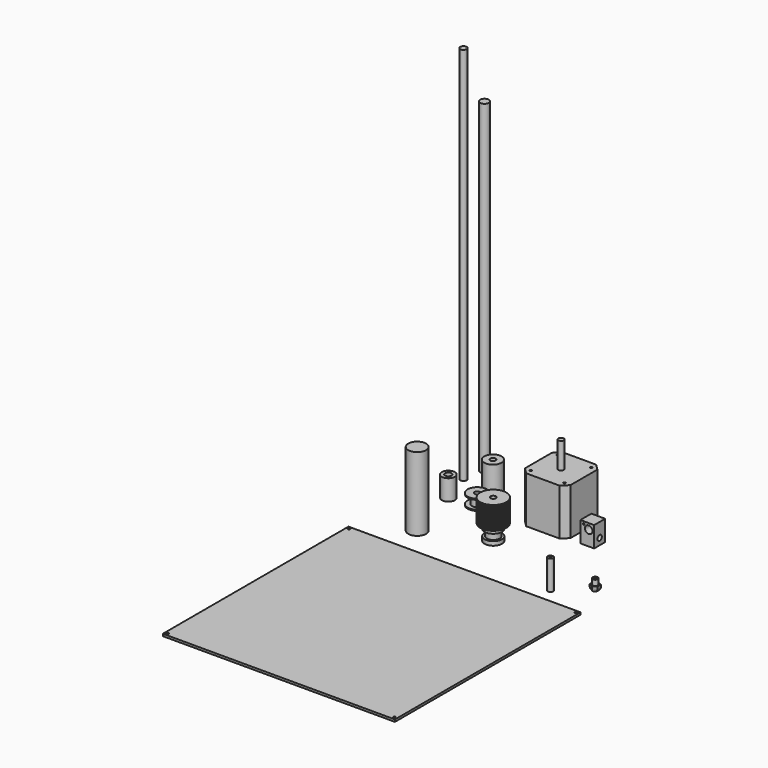
from build123d import *

# Parameters (mm, degrees)
F0_R         = 3
F1_DEPTH     = 350
F2_R         = 8
F2_R_2       = 4
F3_DEPTH     = 25
F4_R         = 6
F4_R_2       = 3
F5_DEPTH     = 19
F6_R         = 5
F7_DEPTH     = 10
F8_R         = 9
F8_R_2       = 5
F9_DEPTH     = 1
F10_R        = 9
F11_DEPTH    = 1
F12_R        = 1
F12_R_2      = 2.5
F13_DEPTH    = 43
F14_DEPTH    = 67
F15_R        = 4
F15_R_2      = 2.5
F16_DEPTH    = 12
F17_R        = 4
F18_DEPTH    = 300
F19_W        = 214
F19_H        = 214
F19_R        = 1
F20_DEPTH    = 2
F21_R        = 8.25
F22_DEPTH    = 68
F23_R        = 2
F24_DEPTH    = 1.7
F25_R        = 8
F25_R_2      = 2
F26_DEPTH    = 3.7
F27_R        = 6
F28_DEPTH    = 6
F29_R        = 8
F29_R_2      = 6
F30_DEPTH    = 3
F31_R        = 4
F32_DEPTH    = 6
F33_R        = 5
F34_DEPTH    = 1.5
F35_R        = 12
F36_DEPTH    = 1
F37_R        = 5
F38_DEPTH    = 1.5
F39_R        = 12
F40_DEPTH    = 1
F41_R        = 5
F42_DEPTH    = 1.5
F43_R        = 12
F44_DEPTH    = 1
F45_R        = 5.5
F46_DEPTH    = 1.5
F47_R        = 12
F48_DEPTH    = 1
F49_R        = 5.5
F50_DEPTH    = 1.5
F51_R        = 12
F52_DEPTH    = 1
F53_R        = 5.5
F54_DEPTH    = 1.5
F55_R        = 12
F56_DEPTH    = 1
F57_R        = 5.5
F58_DEPTH    = 1.5
F59_R        = 12
F60_DEPTH    = 1
F61_R        = 5.5
F62_DEPTH    = 1.5
F63_R        = 12
F64_DEPTH    = 1
F65_R        = 5.5
F66_DEPTH    = 1.5
F67_R        = 12
F67_R_2      = 5.5
F68_DEPTH    = 1
F69_R        = 0.875
F70_DEPTH    = 63
F71_R        = 2.5
F71_R_2      = 0.875
F72_DEPTH    = 15
F73_W        = 12.7
F73_H        = 19
F73_R        = 0.75
F73_R_2      = 3.5
F74_DEPTH    = 12.7
F75_R        = 2.5
F76_DEPTH    = 25
F77_R        = 0.1
F78_DEPTH    = 5
F79_T1_DEPTH = 19.975261396
F79_T3_DEPTH = 19.975261396
F79_T5_DEPTH = 19.975261396
F79_T7_DEPTH = 19.975261396
F79_T9_DEPTH = 19.975261396
F80_R        = 0.875
F81_DEPTH    = 3.04
F82_R        = 2.5
F82_R_2      = 0.875
F83_DEPTH    = 5
F84_R        = 2.5
F84_R_2      = 0.875
F85_DEPTH    = 27
F86_R        = 2.5
F87_DEPTH    = 25


# Not quite as in the source:
# - a fillet or chamfer that OpenCascade refuses, or shapes differently, is made with other operations: its cross-section is extruded or revolved along the edge and cut away or added


with BuildPart() as f1:
    # F0 (on Top) → F1 (new body)
    with BuildSketch(Plane.XY):
        with Locations((-57.2636425495, 36.8765890598)):
            Circle(F0_R)
    extrude(amount=F1_DEPTH)


with BuildPart() as f3:
    # F2 (on Top) → F3 (new body)
    with BuildSketch(Plane.XY):
        with Locations((-29.7810900956, 36.4768393338)):
            Circle(F2_R)
        with Locations((-29.7810900956, 36.4768393338)):
            Circle(F2_R_2, mode=Mode.SUBTRACT)
    extrude(amount=F3_DEPTH)

    # F15 (on face) → F16 (join)
    with BuildSketch(Plane.XY.offset(25)):
        with Locations((-29.7810900956, 36.4768393338)):
            Circle(F15_R)
        with Locations((-29.7810900956, 36.4768393338)):
            Circle(F15_R_2, mode=Mode.SUBTRACT)
    extrude(amount=-F16_DEPTH)


with BuildPart() as f5:
    # F4 (on Top) → F5 (new body)
    with BuildSketch(Plane.XY):
        with Locations((-47.5174151361, 7.268529851)):
            Circle(F4_R)
        with Locations((-47.5174151361, 7.268529851)):
            Circle(F4_R_2, mode=Mode.SUBTRACT)
    extrude(amount=F5_DEPTH)


with BuildPart() as f7:
    # F6 (on Top) → F7 (new body)
    with BuildSketch(Plane.XY):
        with Locations((-24.0222588181, 11.2928301096)):
            Circle(F6_R)
    extrude(amount=F7_DEPTH)

    # F8 (on face) → F9 (join)
    with BuildSketch(Plane.XY.offset(10)):
        with Locations((-24.0222588181, 11.2928301096)):
            Circle(F8_R)
        with Locations((-24.0222588181, 11.2928301096)):
            Circle(F8_R_2, mode=Mode.SUBTRACT)
    extrude(amount=-F9_DEPTH)

    # F10 (on face) → F11 (join)
    with BuildSketch(Plane(origin=(0, 0, 0), x_dir=(1, 0, 0), z_dir=(0, 0, -1))):
        with Locations((-24.0552949804, -11.3842185209)):
            Circle(F10_R)
    extrude(amount=-F11_DEPTH)

    # F86 (on face) → F87 (cut)
    with BuildSketch(Plane.XY.offset(10)):
        with Locations((-24.0222588181, 11.2928301096)):
            Circle(F86_R)
    extrude(amount=-F87_DEPTH, mode=Mode.SUBTRACT)


with BuildPart() as f13:
    # F12 (on Top) → F13 (new body)
    with BuildSketch(Plane.XY):
        Polygon((54.8616796434, 49.6951151714), (23.8616796434, 49.6951151714), (18.3616796434, 44.1951151714), (18.3616796434, 13.1951151714), (23.8616796434, 7.6951151714), (54.8616796434, 7.6951151714), (60.3616796434, 13.1951151714), (60.3616796434, 44.1951151714), align=None)
        with Locations((23.8616796434, 13.1951151714)):
            Circle(F12_R, mode=Mode.SUBTRACT)
        with Locations((54.8616796434, 13.1951151714)):
            Circle(F12_R, mode=Mode.SUBTRACT)
        with Locations((23.8616796434, 44.1951151714)):
            Circle(F12_R, mode=Mode.SUBTRACT)
        with Locations((39.3616796434, 28.6951151714)):
            Circle(F12_R_2, mode=Mode.SUBTRACT)
        with Locations((54.8616796434, 44.1951151714)):
            Circle(F12_R, mode=Mode.SUBTRACT)
    extrude(amount=F13_DEPTH)

    # F12 (on Top) → F14 (join)
    with BuildSketch(Plane.XY):
        with Locations((39.3616796434, 28.6951151714)):
            Circle(F12_R_2)
    extrude(amount=F14_DEPTH)


with BuildPart() as f18:
    # F17 (on Top) → F18 (new body)
    with BuildSketch(Plane.XY):
        with Locations((-53.5317584872, 56.4855635166)):
            Circle(F17_R)
    extrude(amount=F18_DEPTH)


with BuildPart() as f20:
    # F19 (on Top) → F20 (new body)
    with BuildSketch(Plane.XY):
        with Locations((33.727236867, -182.6495461464)):
            Rectangle(F19_W, F19_H)
        with Locations((-70.772763133, -287.1495461464)):
            Circle(F19_R, mode=Mode.SUBTRACT)
        with Locations((138.227236867, -287.1495461464)):
            Circle(F19_R, mode=Mode.SUBTRACT)
        with Locations((-70.772763133, -78.1495461464)):
            Circle(F19_R, mode=Mode.SUBTRACT)
        with Locations((138.227236867, -78.1495461464)):
            Circle(F19_R, mode=Mode.SUBTRACT)
    extrude(amount=F20_DEPTH)


with BuildPart() as f22:
    # F21 (on Top) → F22 (new body)
    with BuildSketch(Plane.XY):
        with Locations((-33.137626946, -46.6584786773)):
            Circle(F21_R)
    extrude(amount=F22_DEPTH)


with BuildPart() as f24:
    # F23 (on Top) → F24 (new body)
    with BuildSketch(Plane.XY):
        with Locations((21.4881356806, -27.2024124861)):
            Circle(F23_R)
    extrude(amount=F24_DEPTH)

    # F25 (on face) → F26 (join)
    with BuildSketch(Plane.XY.offset(1.7)):
        with Locations((21.4881356806, -27.2024124861)):
            Circle(F25_R)
        with Locations((21.4881356806, -27.2024124861)):
            Circle(F25_R_2, mode=Mode.SUBTRACT)
        with Locations((21.4881356806, -27.2024124861)):
            Circle(F25_R_2)
    extrude(amount=F26_DEPTH)

    # F27 (on face) → F28 (join)
    with BuildSketch(Plane.XY.offset(5.4)):
        with Locations((21.4881356806, -27.2024124861)):
            Circle(F27_R)
    extrude(amount=F28_DEPTH)

    # F29 (on face) → F30 (join)
    with BuildSketch(Plane.XY.offset(11.4)):
        with Locations((21.4881356806, -27.2024124861)):
            Circle(F29_R)
        with Locations((21.4881356806, -27.2024124861)):
            Circle(F29_R_2, mode=Mode.SUBTRACT)
        with Locations((21.4881356806, -27.2024124861)):
            Circle(F29_R_2)
    extrude(amount=F30_DEPTH)

    # F31 (on face) → F32 (cut)
    with BuildSketch(Plane(origin=(0, 0, 0), x_dir=(1, 0, 0), z_dir=(0, 0, -1))):
        with Locations((21.4881356806, 27.2024124861)):
            Circle(F31_R)
    extrude(amount=-F32_DEPTH, mode=Mode.SUBTRACT)

    # F33 (on face) → F34 (join)
    with BuildSketch(Plane.XY.offset(14.4)):
        with Locations((21.4881356806, -27.2024124861)):
            Circle(F33_R)
    extrude(amount=F34_DEPTH)

    # F35 (on face) → F36 (join)
    with BuildSketch(Plane.XY.offset(15.9)):
        with Locations((21.4881356806, -27.2024124861)):
            Circle(F35_R)
    extrude(amount=F36_DEPTH)

    # F37 (on face) → F38 (join)
    with BuildSketch(Plane.XY.offset(16.9)):
        with Locations((21.4881356806, -27.2024124861)):
            Circle(F37_R)
    extrude(amount=F38_DEPTH)

    # F39 (on face) → F40 (join)
    with BuildSketch(Plane.XY.offset(18.4)):
        with Locations((21.4881356806, -27.2024124861)):
            Circle(F39_R)
    extrude(amount=F40_DEPTH)

    # F41 (on face) → F42 (join)
    with BuildSketch(Plane.XY.offset(19.4)):
        with Locations((21.4881356806, -27.2024124861)):
            Circle(F41_R)
    extrude(amount=F42_DEPTH)

    # F43 (on face) → F44 (join)
    with BuildSketch(Plane.XY.offset(20.9)):
        with Locations((21.4881356806, -27.2024124861)):
            Circle(F43_R)
    extrude(amount=F44_DEPTH)

    # F45 (on face) → F46 (join)
    with BuildSketch(Plane.XY.offset(21.9)):
        with Locations((21.4881356806, -27.2024124861)):
            Circle(F45_R)
    extrude(amount=F46_DEPTH)

    # F47 (on face) → F48 (join)
    with BuildSketch(Plane.XY.offset(23.4)):
        with Locations((21.4881356806, -27.2024124861)):
            Circle(F47_R)
    extrude(amount=F48_DEPTH)

    # F49 (on face) → F50 (join)
    with BuildSketch(Plane.XY.offset(24.4)):
        with Locations((21.4881356806, -27.2024124861)):
            Circle(F49_R)
    extrude(amount=F50_DEPTH)

    # F51 (on face) → F52 (join)
    with BuildSketch(Plane.XY.offset(25.9)):
        with Locations((21.4881356806, -27.2024124861)):
            Circle(F51_R)
    extrude(amount=F52_DEPTH)

    # F53 (on face) → F54 (join)
    with BuildSketch(Plane.XY.offset(26.9)):
        with Locations((21.4881356806, -27.2024124861)):
            Circle(F53_R)
    extrude(amount=F54_DEPTH)

    # F55 (on face) → F56 (join)
    with BuildSketch(Plane.XY.offset(28.4)):
        with Locations((21.4881356806, -27.2024124861)):
            Circle(F55_R)
    extrude(amount=F56_DEPTH)

    # F57 (on face) → F58 (join)
    with BuildSketch(Plane.XY.offset(29.4)):
        with Locations((21.4881356806, -27.2024124861)):
            Circle(F57_R)
    extrude(amount=F58_DEPTH)

    # F59 (on face) → F60 (join)
    with BuildSketch(Plane.XY.offset(30.9)):
        with Locations((21.4881356806, -27.2024124861)):
            Circle(F59_R)
    extrude(amount=F60_DEPTH)

    # F61 (on face) → F62 (join)
    with BuildSketch(Plane.XY.offset(31.9)):
        with Locations((21.4881356806, -27.2024124861)):
            Circle(F61_R)
    extrude(amount=F62_DEPTH)

    # F63 (on face) → F64 (join)
    with BuildSketch(Plane.XY.offset(33.4)):
        with Locations((21.4881356806, -27.2024124861)):
            Circle(F63_R)
    extrude(amount=F64_DEPTH)

    # F65 (on face) → F66 (join)
    with BuildSketch(Plane.XY.offset(34.4)):
        with Locations((21.4881356806, -27.2024124861)):
            Circle(F65_R)
    extrude(amount=F66_DEPTH)

    # F67 (on face) → F68 (join)
    with BuildSketch(Plane.XY.offset(35.9)):
        with Locations((21.4881356806, -27.2024124861)):
            Circle(F67_R)
        with Locations((21.4881356806, -27.2024124861)):
            Circle(F67_R_2, mode=Mode.SUBTRACT)
        with Locations((21.4881356806, -27.2024124861)):
            Circle(F67_R_2)
    extrude(amount=F68_DEPTH)

    # F69 (on face) → F70 (cut)
    with BuildSketch(Plane(origin=(0, 0, 6), x_dir=(1, 0, 0), z_dir=(0, 0, -1))):
        with Locations((21.4881356806, 27.2024124861)):
            Circle(F69_R)
    extrude(amount=-F70_DEPTH, mode=Mode.SUBTRACT)

    # F71 (on face) → F72 (cut)
    with BuildSketch(Plane.XY.offset(36.9)):
        with Locations((21.4881356806, -27.2024124861)):
            Circle(F71_R)
        with Locations((21.4881356806, -27.2024124861)):
            Circle(F71_R_2, mode=Mode.SUBTRACT)
    extrude(amount=-F72_DEPTH, mode=Mode.SUBTRACT)


with BuildPart() as f74:
    # F73 (on Front) → F74 (new body)
    with BuildSketch(Plane.XZ):
        with Locations((96.546877718, 25.4235037863)):
            Rectangle(F73_W, F73_H)
        with Locations((93.1878611445, 32.6125212014)):
            Circle(F73_R, mode=Mode.SUBTRACT)
        with Locations((97.896877718, 29.5235037863)):
            Circle(F73_R_2, mode=Mode.SUBTRACT)
    extrude(amount=F74_DEPTH)

    # F75 (on face) → F76 (cut)
    with BuildSketch(Plane(origin=(90.196877718, 0, 0), x_dir=(0, -1, 0), z_dir=(-1, 0, 0))):
        with Locations((6.35, 21.9235037863)):
            Circle(F75_R)
    extrude(amount=-F76_DEPTH, mode=Mode.SUBTRACT)


with BuildPart() as f78:
    # F77 (on Top) → F78 (new body)
    with BuildSketch(Plane.XY):
        Polygon((121.874764204, -37.4743435914), (121.874764204, -41.5157954758), (125.374764204, -43.5365214179), (128.874764204, -41.5157954758), (128.874764204, -37.4743435914), (125.374764204, -35.4536176493), align=None)
        with Locations((125.374764204, -39.4950695336)):
            Circle(F77_R, mode=Mode.SUBTRACT)
    extrude(amount=F78_DEPTH)

    # F79: fillet of radius 3.1867619023 on 6 edges, made by hand

    # F79_s2 → F79_t1 (cut)
    with BuildSketch(Plane(origin=(85.5787482909, 49.4089133627, 0), x_dir=(0, 0, 1), z_dir=(-0.8660254038, -0.5, 0))):
        with BuildLine():
            add(Edge.make_bspline(
                [(3.1867619023, -93.3911156423), (0, -93.3911156423), (0, -96.5778775447)],
                knots=[0, 0, 0, 1, 1, 1], degree=2, weights=[1, 1, 1]))
            Line((0, -96.5778775447), (0, -93.3911156423))
            Line((0, -93.3911156423), (3.1867619023, -93.3911156423))
        make_face()
    extrude(amount=F79_T1_DEPTH, mode=Mode.SUBTRACT)

    # F79_s4 → F79_t3 (cut)
    with BuildSketch(Plane.XZ.offset(29.5074388356)):
        with BuildLine():
            add(Edge.make_bspline(
                [(121.874764204, 3.1867619023), (121.874764204, 0), (125.0615261064, 0)],
                knots=[0, 0, 0, 1, 1, 1], degree=2, weights=[1, 1, 1]))
            Line((125.0615261064, 0), (121.874764204, 0))
            Line((121.874764204, 0), (121.874764204, 3.1867619023))
        make_face()
        with BuildLine():
            add(Edge.make_bspline(
                [(128.874764204, 3.1867619023), (128.874764204, 0), (125.6880023017, 0)],
                knots=[0, 0, 0, 1, 1, 1], degree=2, weights=[1, 1, 1]))
            Line((125.6880023017, 0), (128.874764204, 0))
            Line((128.874764204, 0), (128.874764204, 3.1867619023))
        make_face()
    extrude(amount=F79_T3_DEPTH, mode=Mode.SUBTRACT)

    # F79_s6 → F79_t5 (cut)
    with BuildSketch(Plane(origin=(119.7824818313, -69.1564481295, 0), x_dir=(0, 0, 1), z_dir=(-0.8660254038, 0.5, 0))):
        with BuildLine():
            add(Edge.make_bspline(
                [(3.1867619023, 31.9836485617), (0, 31.9836485617), (0, 28.7968866594)],
                knots=[0, 0, 0, 1, 1, 1], degree=2, weights=[1, 1, 1]))
            Line((0, 28.7968866594), (0, 31.9836485617))
            Line((0, 31.9836485617), (3.1867619023, 31.9836485617))
        make_face()
    extrude(amount=F79_T5_DEPTH, mode=Mode.SUBTRACT)

    # F79_s8 → F79_t7 (cut)
    with BuildSketch(Plane(origin=(68.2796644748, 39.4212826647, 0), x_dir=(0, 0, 1), z_dir=(0.8660254038, 0.5, 0))):
        with BuildLine():
            add(Edge.make_bspline(
                [(3.1867619023, 100.3911156423), (0, 100.3911156423), (0, 97.20435374)],
                knots=[0, 0, 0, 1, 1, 1], degree=2, weights=[1, 1, 1]))
            Line((0, 97.20435374), (0, 100.3911156423))
            Line((0, 100.3911156423), (3.1867619023, 100.3911156423))
        make_face()
    extrude(amount=F79_T7_DEPTH, mode=Mode.SUBTRACT)

    # F79_s10 → F79_t9 (cut)
    with BuildSketch(Plane(origin=(102.4833980151, -59.1688174315, 0), x_dir=(0, 0, 1), z_dir=(0.8660254038, -0.5, 0))):
        with BuildLine():
            add(Edge.make_bspline(
                [(3.1867619023, -24.9836485617), (0, -24.9836485617), (0, -28.170410464)],
                knots=[0, 0, 0, 1, 1, 1], degree=2, weights=[1, 1, 1]))
            Line((0, -28.170410464), (0, -24.9836485617))
            Line((0, -24.9836485617), (3.1867619023, -24.9836485617))
        make_face()
    extrude(amount=F79_T9_DEPTH, mode=Mode.SUBTRACT)

    # F80 (on face) → F81 (cut)
    with BuildSketch(Plane.XY.offset(5)):
        with Locations((125.374764204, -39.4950695336)):
            Circle(F80_R)
    extrude(amount=-F81_DEPTH, mode=Mode.SUBTRACT)

    # F82 (on face) → F83 (join)
    with BuildSketch(Plane.XY.offset(5)):
        with Locations((125.374764204, -39.4950695336)):
            Circle(F82_R)
        with Locations((125.374764204, -39.4950695336)):
            Circle(F82_R_2, mode=Mode.SUBTRACT)
    extrude(amount=F83_DEPTH)


with BuildPart() as f85:
    # F84 (on Top) → F85 (new body)
    with BuildSketch(Plane.XY):
        with Locations((100.0474393368, -59.4899617136)):
            Circle(F84_R)
        with Locations((100.0474393368, -59.4899617136)):
            Circle(F84_R_2, mode=Mode.SUBTRACT)
    extrude(amount=F85_DEPTH)


solid = Compound([f1.part, f3.part, f5.part, f7.part, f13.part, f18.part, f20.part, f22.part, f24.part, f74.part, f78.part, f85.part])
